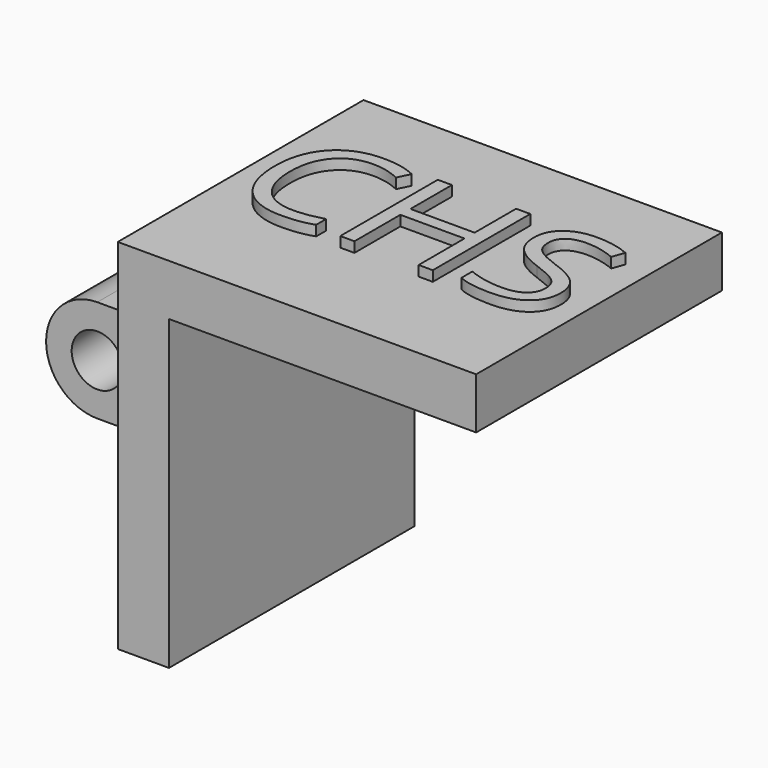
from build123d import *

# Parameters (mm, degrees)
F1_DEPTH     = 19.05
F2_W         = 12.7
F2_H         = 12.7
F3_DEPTH     = 19.05
F5_R         = 6.34999
F4_R         = 3.175
F6_DEPTH     = 25.4
F7_TEXT_SIZE = 21.1666666667
F8_DEPTH     = 1.27


# Not quite as in the source:
# - a fillet or chamfer is up to 0.001 mm smaller than in the source, because OpenCascade refuses the exact size
# - a feature names something its author has since deleted; it is built from what else it names
# - Text() gives the source's letters only with a copy of the font that has no kerning and outlines rounded to 1/6400 em; it was checked with that copy


with BuildPart() as f1:
    # F0 (on Front) → F1 (new body, symmetric)
    with BuildSketch(Plane.XZ):
        Polygon((22.225, 22.225), (-22.225, 22.225), (-22.225, -22.225), (-15.875, -22.225), (-15.875, 15.875), (22.225, 15.875), align=None)
    extrude(amount=F1_DEPTH, both=True)

    # F2 (on face) → F3 (join)
    with BuildSketch(Plane(origin=(-22.225, 0, 0), x_dir=(0, -1, 0), z_dir=(-1, 0, 0))):
        Rectangle(F2_W, F2_H)
    extrude(amount=F3_DEPTH)

    # F5 (radius 6.35 in the source; OpenCascade refuses exactly that, so slightly less here)
    f5_edges = [f1.edges().sort_by_distance(p)[0] for p in [
        (-41.275, 0, 6.35),
        (-41.275, 0, -6.35),
    ]]
    fillet(f5_edges, radius=F5_R)

    # F4 (on face) → F6 (cut)
    with BuildSketch(Plane.XZ.offset(6.35)):
        with Locations((-34.925, 0)):
            Circle(F4_R)
    extrude(amount=-F6_DEPTH, mode=Mode.SUBTRACT)

    # F7 (on face) → F8 (join)
    with BuildSketch(Plane.XY.offset(22.225)):
        with Locations((-20.0743616509, -6.5282654488)):
            Text('CHS', F7_TEXT_SIZE, font='Open Sans', text_align=(TextAlign.LEFT, TextAlign.BOTTOM))
    extrude(amount=F8_DEPTH)


solid = f1.part
